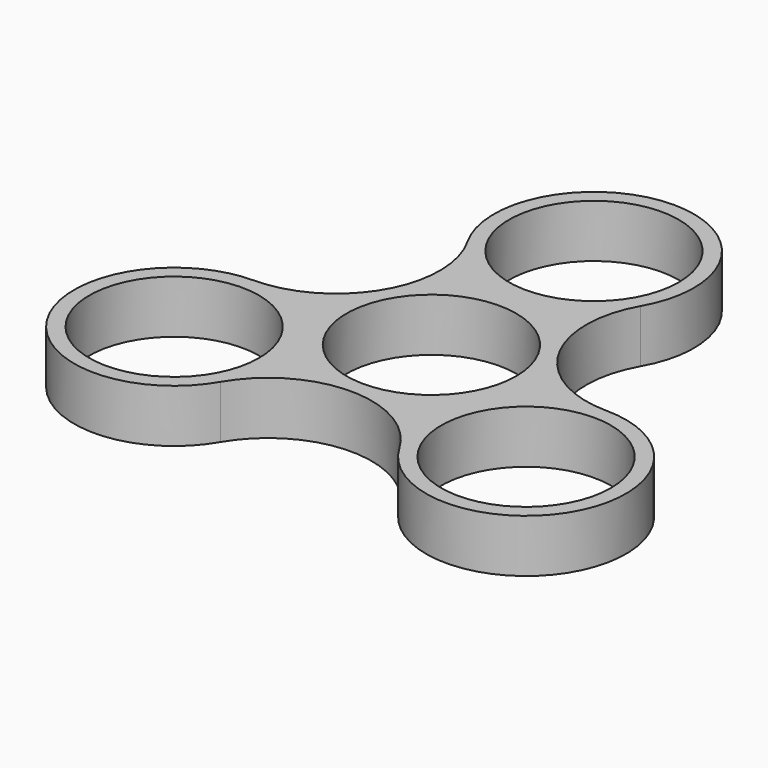
from build123d import *

# Parameters (mm, degrees)
F0_R     = 11.2
F1_DEPTH = 7


# Not quite as in the source:
# - ends of sketch curves that miss each other by under 0.0002 mm in the source are joined


with BuildPart() as f1:
    # F0 (on Top) → F1 (new body)
    with BuildSketch(Plane.XY):
        with BuildLine():
            ThreePointArc((23.1851437088, -0.209827322), (11.4809905002, 6.6524743946), (11.4315817283, 20.219933477))
            ThreePointArc((11.4315817283, 20.219933477), (-9.27972e-05, 40.0198531118), (-11.4314889311, 20.2197727475))
            ThreePointArc((-11.4314889311, 20.2197727475), (-11.4807071504, 6.6523126094), (-23.1847645001, -0.2101533167))
            ThreePointArc((-23.1847645001, -0.2101533167), (-29.8083976459, -1.968183302), (-34.65797177, -6.8101680495))
            ThreePointArc((-34.65797177, -6.8101680495), (-29.8265597828, -24.8415250127), (-11.7950971191, -20.0105075285))
            ThreePointArc((-11.7950971191, -20.0105075285), (0.0002818311, -13.2693854266), (11.7957555615, -20.0103416826))
            ThreePointArc((11.7957555615, -20.0103416826), (29.8270373154, -24.8412493104), (34.6587334239, -6.8101809539))
            ThreePointArc((34.6587334239, -6.8101809539), (29.8271641279, -1.9786795899), (23.2271516953, -0.2102613183))
            ThreePointArc((23.2271516953, -0.2102613183), (23.2061475356, -0.2100604335), (23.1851437088, -0.209827322))
        make_face()
        with Locations((-23.2263900417, -13.4100876845)):
            Circle(F0_R, mode=Mode.SUBTRACT)
        Circle(F0_R, mode=Mode.SUBTRACT)
        with Locations((23.2269557018, -13.4097611005)):
            Circle(F0_R, mode=Mode.SUBTRACT)
        with Locations((0, 26.8198531121)):
            Circle(F0_R, mode=Mode.SUBTRACT)
        with BuildLine():
            ThreePointArc((34.6587334239, -6.8101809539), (29.8090523924, -1.9679079658), (23.1851437088, -0.209827322))
            ThreePointArc((23.1851437088, -0.209827322), (23.2061475356, -0.2100604335), (23.2271516953, -0.2102613183))
            ThreePointArc((23.2271516953, -0.2102613183), (29.8271641279, -1.9786795899), (34.6587334239, -6.8101809539))
        make_face()
        with BuildLine():
            ThreePointArc((11.7957555615, -20.0103416826), (29.8273248569, -24.8417502492), (34.6587334239, -6.8101809539))
            ThreePointArc((34.6587334239, -6.8101809539), (29.8270373154, -24.8412493104), (11.7957555615, -20.0103416826))
        make_face()
        with BuildLine():
            ThreePointArc((-11.7950971191, -20.0105075285), (-29.8265597828, -24.8415250127), (-34.65797177, -6.8101680495))
            ThreePointArc((-34.65797177, -6.8101680495), (-29.8268485884, -24.8420252217), (-11.7950971191, -20.0105075285))
        make_face()
    extrude(amount=F1_DEPTH)


solid = f1.part
